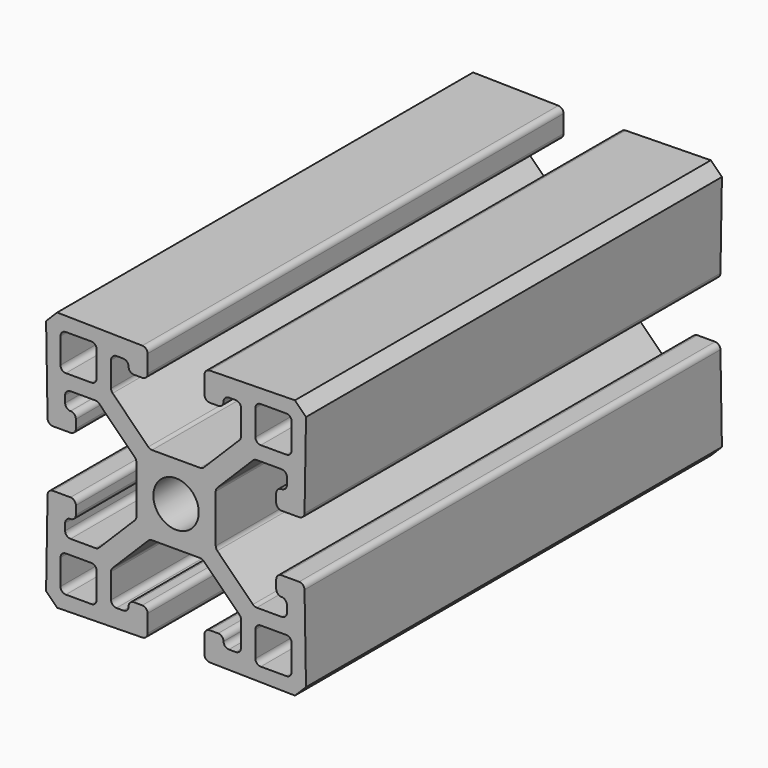
from build123d import *

# Parameters (mm, degrees)
F1_DEPTH = 76.2


# Not quite as in the source:
# - ends of sketch curves that miss each other by under 0.0002 mm in the source are joined


with BuildPart() as f1:
    # F0 (on Front) → F1 (new body)
    with BuildSketch(Plane.XZ):
        with BuildLine():
            Line((-55.0240708, -0.2623312), (-56.2432962, -0.2623312))
            ThreePointArc((-56.2432962, -0.2623312), (-56.8000720795, -0.4929553205), (-57.0306962, -1.0497312))
            ThreePointArc((-57.0306962, -1.0497312), (-57.2613457205, -1.6065070795), (-57.8181216, -1.8371312))
            Line((-57.8181216, -1.8371312), (-58.8087216, -1.8371312))
            ThreePointArc((-58.8087216, -1.8371312), (-59.3654974795, -1.6065070795), (-59.5961216, -1.0497312))
            Line((-59.5961216, -1.0497312), (-59.596147, 2.5921208))
            ThreePointArc((-59.596147, 2.5921208), (-59.5361843439, 2.8934457346), (-59.3654974795, 3.1488966795))
            Line((-59.3654974795, 3.1488966795), (-54.14264, 8.3717892))
            ThreePointArc((-54.14264, 8.3717892), (-53.8871715346, 8.5424585439), (-53.5858466, 8.6023958))
            Line((-53.5858466, 8.6023958), (-46.556168, 8.6023958))
            ThreePointArc((-46.556168, 8.6023958), (-46.2548430654, 8.5424585439), (-45.9993921205, 8.3717716795))
            Line((-45.9993921205, 8.3717716795), (-40.7764996, 3.1488888))
            ThreePointArc((-40.7764996, 3.1488888), (-40.6058048561, 2.8934457346), (-40.5458676, 2.5921208))
            Line((-40.5458676, 2.5921208), (-40.5458676, -1.0497312))
            ThreePointArc((-40.5458676, -1.0497312), (-40.7764917205, -1.6065070795), (-41.3332676, -1.8371312))
            Line((-41.3332676, -1.8371312), (-42.323893, -1.8371312))
            ThreePointArc((-42.323893, -1.8371312), (-42.8806688795, -1.6065070795), (-43.111293, -1.0497312))
            ThreePointArc((-43.111293, -1.0497312), (-43.3419425205, -0.4929553205), (-43.8987184, -0.2623312))
            Line((-43.8987184, -0.2623312), (-45.1179184, -0.2623312))
            ThreePointArc((-45.1179184, -0.2623312), (-45.6746942795, -0.4929553205), (-45.9053184, -1.0497312))
            Line((-45.9053184, -1.0497312), (-45.9053438, -3.6259516))
            ThreePointArc((-45.9053438, -3.6259516), (-45.679531628, -4.1778477335), (-45.1316599236, -4.4132316839))
            Line((-45.1316599236, -4.4132316839), (-32.646366, -4.631182))
            Line((-32.646366, -4.631182), (-31.0207406, -3.0055566))
            Line((-31.0207406, -3.0055566), (-31.2386726, 9.4797626))
            ThreePointArc((-31.2386726, 9.4797626), (-31.4740494665, 10.027634428), (-32.0259456, 10.2534212))
            Line((-32.0259456, 10.2534212), (-34.6021914, 10.2534212))
            ThreePointArc((-34.6021914, 10.2534212), (-35.1589672795, 10.0227970795), (-35.3895914, 9.4660212))
            Line((-35.3895914, 9.4660212), (-35.3895914, 8.2467958))
            ThreePointArc((-35.3895914, 8.2467958), (-35.1589672795, 7.6900199205), (-34.6021914, 7.4593958))
            ThreePointArc((-34.6021914, 7.4593958), (-34.0454155205, 7.2287462795), (-33.8147914, 6.6719704))
            Line((-33.8147914, 6.6719704), (-33.814766, 5.6813704))
            ThreePointArc((-33.814766, 5.6813704), (-34.0454155205, 5.1245945205), (-34.6021914, 4.8939704))
            Line((-34.6021914, 4.8939704), (-38.244018, 4.893945))
            ThreePointArc((-38.244018, 4.893945), (-38.5453429346, 4.9539076561), (-38.8007938795, 5.1245945205))
            Line((-38.8007938795, 5.1245945205), (-44.0236864, 10.347452))
            ThreePointArc((-44.0236864, 10.347452), (-44.1943811439, 10.6029204654), (-44.2543184, 10.9042454))
            Line((-44.2543184, 10.9042454), (-44.2543184, 17.933924))
            ThreePointArc((-44.2543184, 17.933924), (-44.1943811439, 18.2352489346), (-44.0236942795, 18.4906998795))
            Line((-44.0236942795, 18.4906998795), (-38.8008114, 23.7135924))
            ThreePointArc((-38.8008114, 23.7135924), (-38.5453429346, 23.8842871439), (-38.244018, 23.9442244))
            Line((-38.244018, 23.9442244), (-34.6021914, 23.9442244))
            ThreePointArc((-34.6021914, 23.9442244), (-34.0454155205, 23.7136002795), (-33.8147914, 23.1568244))
            Line((-33.8147914, 23.1568244), (-33.814766, 22.166199))
            ThreePointArc((-33.814766, 22.166199), (-34.0454155205, 21.6094231205), (-34.6021914, 21.378799))
            ThreePointArc((-34.6021914, 21.378799), (-35.1589672795, 21.1481494795), (-35.3895914, 20.5913736))
            Line((-35.3895914, 20.5913736), (-35.3895914, 19.3721482))
            ThreePointArc((-35.3895914, 19.3721482), (-35.1589672795, 18.8153723205), (-34.6021914, 18.5847482))
            Line((-34.6021914, 18.5847482), (-32.0259456, 18.5847482))
            ThreePointArc((-32.0259456, 18.5847482), (-31.4740494665, 18.810534972), (-31.2386655161, 19.3584066764))
            Line((-31.2386655161, 19.3584066764), (-31.0207406, 31.843726))
            Line((-31.0207406, 31.843726), (-32.646366, 33.4693514))
            Line((-32.646366, 33.4693514), (-45.1316852, 33.2514194))
            ThreePointArc((-45.1316852, 33.2514194), (-45.679531628, 33.0160425335), (-45.9053184, 32.4641464))
            Line((-45.9053184, 32.4641464), (-45.9053438, 29.8879006))
            ThreePointArc((-45.9053438, 29.8879006), (-45.6746942795, 29.3311247205), (-45.1179184, 29.1005006))
            Line((-45.1179184, 29.1005006), (-43.8987184, 29.1005006))
            ThreePointArc((-43.8987184, 29.1005006), (-43.3419425205, 29.3311247205), (-43.1113184, 29.8879006))
            ThreePointArc((-43.1113184, 29.8879006), (-42.8806688795, 30.4446764795), (-42.323893, 30.6753006))
            Line((-42.323893, 30.6753006), (-41.3332676, 30.675326))
            ThreePointArc((-41.3332676, 30.675326), (-40.7764917205, 30.4446764795), (-40.5458676, 29.8879006))
            Line((-40.5458676, 29.8879006), (-40.5458676, 26.246074))
            ThreePointArc((-40.5458676, 26.246074), (-40.6058048561, 25.9447490654), (-40.7764917205, 25.6892981205))
            Line((-40.7764917205, 25.6892981205), (-45.9993746, 20.4664056))
            ThreePointArc((-45.9993746, 20.4664056), (-46.2548430654, 20.2957108561), (-46.556168, 20.2357736))
            Line((-46.556168, 20.2357736), (-53.5858466, 20.2357736))
            ThreePointArc((-53.5858466, 20.2357736), (-53.8871715346, 20.2957108561), (-54.1426224795, 20.4663977205))
            Line((-54.1426224795, 20.4663977205), (-59.365515, 25.6892806))
            ThreePointArc((-59.365515, 25.6892806), (-59.5361843439, 25.9447490654), (-59.5961216, 26.246074))
            Line((-59.5961216, 26.246074), (-59.596147, 29.8879006))
            ThreePointArc((-59.596147, 29.8879006), (-59.3654974795, 30.4446764795), (-58.8087216, 30.6753006))
            Line((-58.8087216, 30.6753006), (-57.8181216, 30.675326))
            ThreePointArc((-57.8181216, 30.675326), (-57.2613457205, 30.4446764795), (-57.0307216, 29.8879006))
            ThreePointArc((-57.0307216, 29.8879006), (-56.8000720795, 29.3311247205), (-56.2432962, 29.1005006))
            Line((-56.2432962, 29.1005006), (-55.0240708, 29.1005006))
            ThreePointArc((-55.0240708, 29.1005006), (-54.4672949205, 29.3311247205), (-54.2366708, 29.8879006))
            Line((-54.2366708, 29.8879006), (-54.2366708, 32.4641464))
            ThreePointArc((-54.2366708, 32.4641464), (-54.462457572, 33.0160425335), (-55.0103292764, 33.2514264839))
            Line((-55.0103292764, 33.2514264839), (-67.4956486, 33.4693514))
            Line((-67.4956486, 33.4693514), (-69.121274, 31.843726))
            Line((-69.121274, 31.843726), (-68.903342, 19.3584068))
            ThreePointArc((-68.903342, 19.3584068), (-68.6679397335, 18.810534972), (-68.1160436, 18.5847482))
            Line((-68.1160436, 18.5847482), (-65.5398232, 18.5847482))
            ThreePointArc((-65.5398232, 18.5847482), (-64.9830473205, 18.8153723205), (-64.7524232, 19.3721482))
            Line((-64.7524232, 19.3721482), (-64.7524232, 20.5913736))
            ThreePointArc((-64.7524232, 20.5913736), (-64.9830473205, 21.1481494795), (-65.5398232, 21.3787736))
            ThreePointArc((-65.5398232, 21.3787736), (-66.0965990795, 21.6094231205), (-66.3272232, 22.166199))
            Line((-66.3272232, 22.166199), (-66.3272232, 23.1568244))
            ThreePointArc((-66.3272232, 23.1568244), (-66.0965990795, 23.7136002795), (-65.5398232, 23.9442244))
            Line((-65.5398232, 23.9442244), (-61.8979712, 23.9442244))
            ThreePointArc((-61.8979712, 23.9442244), (-61.5966462654, 23.8842871439), (-61.3411953205, 23.7136002795))
            Line((-61.3411953205, 23.7136002795), (-56.1183028, 18.4907174))
            ThreePointArc((-56.1183028, 18.4907174), (-55.9476334561, 18.2352489346), (-55.8876962, 17.933924))
            Line((-55.8876962, 17.933924), (-55.8876962, 10.9042454))
            ThreePointArc((-55.8876962, 10.9042454), (-55.9476334561, 10.6029204654), (-56.1183203205, 10.3474695205))
            Line((-56.1183203205, 10.3474695205), (-61.3412032, 5.124577))
            ThreePointArc((-61.3412032, 5.124577), (-61.5966462654, 4.9539076561), (-61.8979712, 4.8939704))
            Line((-61.8979712, 4.8939704), (-65.5398232, 4.893945))
            ThreePointArc((-65.5398232, 4.893945), (-66.0965990795, 5.1245945205), (-66.3272232, 5.6813704))
            Line((-66.3272232, 5.6813704), (-66.3272232, 6.6719704))
            ThreePointArc((-66.3272232, 6.6719704), (-66.0965990795, 7.2287462795), (-65.5398232, 7.4593704))
            ThreePointArc((-65.5398232, 7.4593704), (-64.9830473205, 7.6900199205), (-64.7524232, 8.2467958))
            Line((-64.7524232, 8.2467958), (-64.7524232, 9.4660212))
            ThreePointArc((-64.7524232, 9.4660212), (-64.9830473205, 10.0227970795), (-65.5398232, 10.2534212))
            Line((-65.5398232, 10.2534212), (-68.1160436, 10.2534212))
            ThreePointArc((-68.1160436, 10.2534212), (-68.6679397335, 10.027634428), (-68.9033236839, 9.4797627236))
            Line((-68.9033236839, 9.4797627236), (-69.121274, -3.0055566))
            Line((-69.121274, -3.0055566), (-67.4956486, -4.631182))
            Line((-67.4956486, -4.631182), (-55.0103294, -4.41325))
            ThreePointArc((-55.0103294, -4.41325), (-54.462457572, -4.1778477335), (-54.2366708, -3.6259516))
            Line((-54.2366708, -3.6259516), (-54.2366708, -1.0497312))
            ThreePointArc((-54.2366708, -1.0497312), (-54.4672949205, -0.4929553205), (-55.0240708, -0.2623312))
        make_face()
        with BuildLine():
            Line((-67.0130486, -1.7355312), (-67.0130486, 1.9983196))
            ThreePointArc((-67.0130486, 1.9983196), (-66.7824154992, 2.5551044597), (-66.2256232, 2.7857195996))
            Line((-66.2256232, 2.7857196), (-62.4917724, 2.7857196))
            ThreePointArc((-62.4917724, 2.7857196), (-61.9349965205, 2.5550954795), (-61.7043724, 1.9983196))
            Line((-61.7043724, 1.9983196), (-61.7043724, -1.7355312))
            ThreePointArc((-61.7043724004, -1.7355312), (-61.9349875403, -2.2923234992), (-62.4917724, -2.5229566))
            Line((-62.4917724, -2.5229566), (-66.2256232, -2.5229566))
            ThreePointArc((-66.2256232, -2.5229566), (-66.78241704, -2.29232504), (-67.0130486, -1.7355312))
        make_face(mode=Mode.SUBTRACT)
        with BuildLine():
            ThreePointArc((-33.1289660004, -1.7355312), (-33.3595811403, -2.2923234992), (-33.916366, -2.5229566))
            Line((-33.916366, -2.5229566), (-37.6502168, -2.5229566))
            ThreePointArc((-37.6502168, -2.5229566), (-38.20701064, -2.29232504), (-38.4376422, -1.7355312))
            Line((-38.4376422, -1.7355312), (-38.4376422, 1.9983196))
            ThreePointArc((-38.4376422, 1.9983196), (-38.2070090992, 2.5551044597), (-37.6502168, 2.7857195996))
            Line((-37.6502168, 2.7857196), (-33.916366, 2.7857196))
            ThreePointArc((-33.916366, 2.7857196), (-33.3595901205, 2.5550954795), (-33.128966, 1.9983196))
            Line((-33.128966, 1.9983196), (-33.128966, -1.7355312))
        make_face(mode=Mode.SUBTRACT)
        with BuildLine():
            Line((-67.0130486, 26.8398752), (-67.0130486, 30.573726))
            ThreePointArc((-67.0130486, 30.573726), (-66.7824154992, 31.1305108597), (-66.2256232, 31.3611259996))
            Line((-66.2256232, 31.361126), (-62.4917724, 31.361126))
            ThreePointArc((-62.4917724, 31.361126), (-61.9349965205, 31.1305018795), (-61.7043724, 30.573726))
            Line((-61.7043724, 30.573726), (-61.7043724, 26.8398752))
            ThreePointArc((-61.7043724004, 26.8398752), (-61.9349875403, 26.2830829008), (-62.4917724, 26.0524498))
            Line((-62.4917724, 26.0524498), (-66.2256232, 26.0524498))
            ThreePointArc((-66.2256232, 26.0524498), (-66.78241704, 26.28308136), (-67.0130486, 26.8398752))
        make_face(mode=Mode.SUBTRACT)
        with BuildLine():
            ThreePointArc((-53.3984454, 14.4190974), (-50.0709946, 17.7465482), (-46.7435438, 14.4190974))
            ThreePointArc((-46.7435438, 14.4190974), (-50.0709946, 11.0916466), (-53.3984454, 14.4190974))
        make_face(mode=Mode.SUBTRACT)
        with BuildLine():
            Line((-33.916366, 26.0524498), (-37.6502168, 26.0524498))
            ThreePointArc((-37.6502168, 26.0524498), (-38.20701064, 26.28308136), (-38.4376422, 26.8398752))
            Line((-38.4376422, 26.8398752), (-38.4376422, 30.573726))
            ThreePointArc((-38.4376422, 30.573726), (-38.2070090992, 31.1305108597), (-37.6502168, 31.3611259996))
            Line((-37.6502168, 31.361126), (-33.916366, 31.361126))
            ThreePointArc((-33.916366, 31.361126), (-33.3595901205, 31.1305018795), (-33.128966, 30.573726))
            Line((-33.128966, 30.573726), (-33.128966, 26.8398752))
            ThreePointArc((-33.1289660004, 26.8398752), (-33.3595811403, 26.2830829008), (-33.916366, 26.0524498))
        make_face(mode=Mode.SUBTRACT)
    extrude(amount=F1_DEPTH)


solid = f1.part
